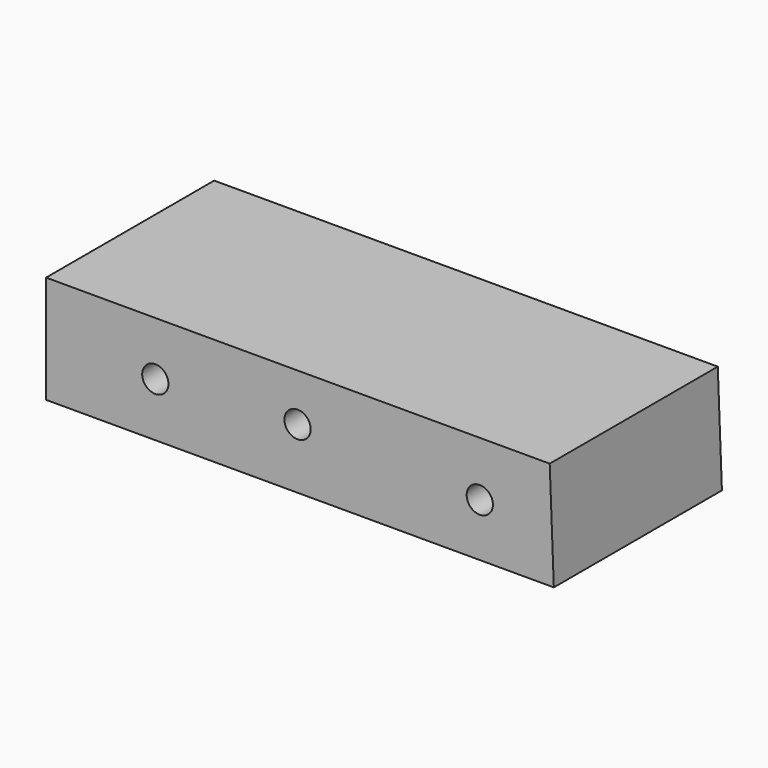
from build123d import *

# Parameters (mm, degrees)
F0_R     = 2.38125
F1_DEPTH = 12.7
F2_DEPTH = 25.4
F3_DEPTH = 25.4
F4_DEPTH = 25.4


# Not quite as in the source:
# - a feature names something its author has since deleted; it is built from what else it names


with BuildPart() as f1:
    # F0 (on Front) → F1 (new body, symmetric)
    with BuildSketch(Plane.XZ):
        Polygon((-45.6028679988, 0), (46.4721320012, 0), (45.7215224688, 19.5158975394), (-45.6028679988, 19.5158975394), align=None)
        with Locations((33.0442860723, 9.6084093675)):
            Circle(F0_R, mode=Mode.SUBTRACT)
        with Locations((-25.7945582271, 9.7579487697)):
            Circle(F0_R, mode=Mode.SUBTRACT)
        with Locations((0, 10.9073175117)):
            Circle(F0_R, mode=Mode.SUBTRACT)
    extrude(amount=F1_DEPTH, both=True)

    # F0 (on Front) → F2 (join)
    with BuildSketch(Plane.XZ):
        Polygon((-45.6028679988, 0), (46.4721320012, 0), (45.7215224688, 19.5158975394), (-45.6028679988, 19.5158975394), align=None)
        with Locations((33.0442860723, 9.6084093675)):
            Circle(F0_R, mode=Mode.SUBTRACT)
        with Locations((-25.7945582271, 9.7579487697)):
            Circle(F0_R, mode=Mode.SUBTRACT)
        with Locations((0, 10.9073175117)):
            Circle(F0_R, mode=Mode.SUBTRACT)
    extrude(amount=F2_DEPTH)

    # F0 (on Front) → F3 (join)
    with BuildSketch(Plane.XZ):
        Polygon((-45.6028679988, 0), (46.4721320012, 0), (45.7215224688, 19.5158975394), (-45.6028679988, 19.5158975394), align=None)
        with Locations((33.0442860723, 9.6084093675)):
            Circle(F0_R, mode=Mode.SUBTRACT)
        with Locations((-25.7945582271, 9.7579487697)):
            Circle(F0_R, mode=Mode.SUBTRACT)
        with Locations((0, 10.9073175117)):
            Circle(F0_R, mode=Mode.SUBTRACT)
    extrude(amount=F3_DEPTH)

    # F0 (on Front) → F4 (join)
    with BuildSketch(Plane.XZ):
        Polygon((-45.6028679988, 0), (46.4721320012, 0), (45.7215224688, 19.5158975394), (-45.6028679988, 19.5158975394), align=None)
        with Locations((33.0442860723, 9.6084093675)):
            Circle(F0_R, mode=Mode.SUBTRACT)
        with Locations((-25.7945582271, 9.7579487697)):
            Circle(F0_R, mode=Mode.SUBTRACT)
        with Locations((0, 10.9073175117)):
            Circle(F0_R, mode=Mode.SUBTRACT)
    extrude(amount=F4_DEPTH)


solid = f1.part
